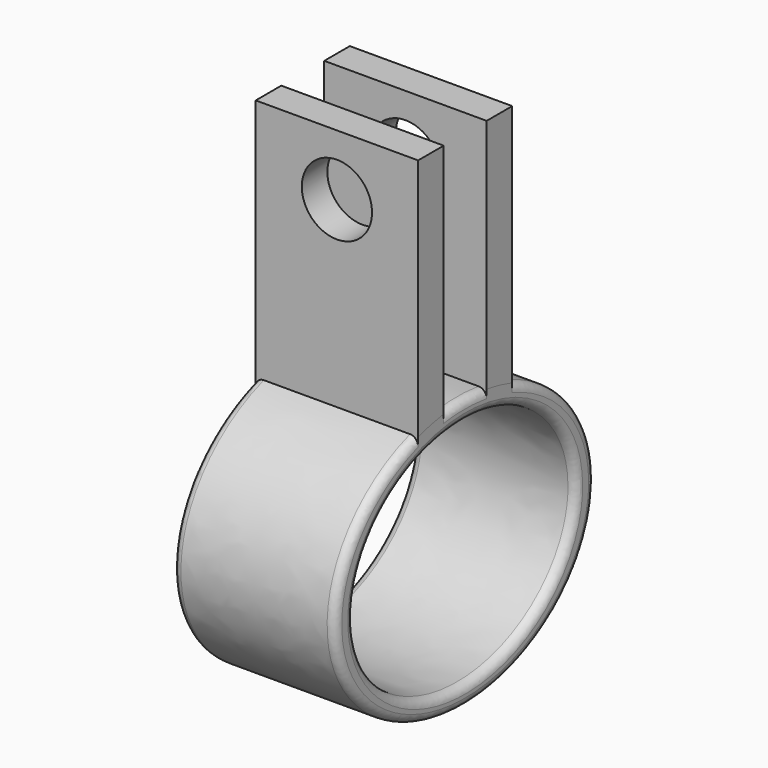
from build123d import *

# Parameters (mm, degrees)
F1_DEPTH = 10.16
F3_DEPTH = 10.16
F4_R     = 2.1971
F5_DEPTH = 25.4
F6_R     = 0.508


with BuildPart() as f1:
    # F0 (on Right) → F1 (new body)
    with BuildSketch(Plane.YZ):
        with BuildLine():
            add(Edge.make_bspline(
                [(10.16, 0), (10.16, 14.6720291858), (-5.08, 7.3360145929), (-20.32, 0), (-5.08, -7.3360145929), (10.16, -14.6720291858), (10.16, 0)],
                knots=[0, 0, 0, 2.0943951024, 2.0943951024, 4.1887902048, 4.1887902048, 6.2831853072, 6.2831853072, 6.2831853072], degree=2, weights=[1, 0.5, 1, 0.5, 1, 0.5, 1]))
        make_face()
        with BuildLine():
            add(Edge.make_bspline(
                [(8.6741, 0), (8.6741, 12.538315796), (-4.33705, 6.269157898), (-17.3482, 0), (-4.33705, -6.269157898), (8.6741, -12.538315796), (8.6741, 0)],
                knots=[0, 0, 0, 2.0943951024, 2.0943951024, 4.1887902048, 4.1887902048, 6.2831853072, 6.2831853072, 6.2831853072], degree=2, weights=[1, 0.5, 1, 0.5, 1, 0.5, 1]))
        make_face(mode=Mode.SUBTRACT)
    extrude(amount=F1_DEPTH)

    # F2 (on face) → F3 (join)
    with BuildSketch(Plane.YZ.offset(10.16)):
        with BuildLine():
            Line((-3.6787074356, 23.1361324366), (-3.6787074356, 7.8961324366))
            add(Edge.make_bspline(
                [(-1.6795329809, 8.3543567658), (-2.7073061404, 8.2107269893), (-3.6787074356, 7.8961324366)],
                knots=[1.698688762, 1.698688762, 1.698688762, 1.9167664316, 1.9167664316, 1.9167664316], degree=2, weights=[0.846760899, 0.8791502713, 0.9223815379]))
            Line((-1.6795329809, 8.3543567658), (-1.6795329809, 23.1361324366))
            Line((-1.6795329809, 23.1361324366), (-3.6787074356, 23.1361324366))
        make_face()
        with BuildLine():
            Line((1.6795329809, 23.1361324366), (1.6795329809, 8.3543567658))
            add(Edge.make_bspline(
                [(3.6787074356, 7.8961324366), (2.7073061404, 8.2107269893), (1.6795329809, 8.3543567658)],
                knots=[1.1863185819, 1.1863185819, 1.1863185819, 1.3749382963, 1.3749382963, 1.3749382963], degree=2, weights=[0.7544123337, 0.7603945573, 0.7744874547]))
            Line((3.6787074356, 7.8961324366), (3.6787074356, 23.1361324366))
            Line((3.6787074356, 23.1361324366), (1.6795329809, 23.1361324366))
        make_face()
    extrude(amount=-F3_DEPTH)

    # F4 (on face) → F5 (cut)
    with BuildSketch(Plane(origin=(0, 3.6787074356, 0), x_dir=(-1, 0, 0), z_dir=(0, 1, 0))):
        with Locations((-5.08, 19.3261324366)):
            Circle(F4_R)
    extrude(amount=-F5_DEPTH, mode=Mode.SUBTRACT)

    # F6
    f6_edges = [f1.edges().sort_by_distance(p)[0] for p in [
        (10.16, -8.6741, 0),
        (10.16, -5.271292, -7.241592),
        (0, -5.271292, -7.241592),
        (0, -8.6741, 0),
        (0, 8.626252, 4.47541),
        (10.16, 8.626252, 4.47541),
        (0, -0.037714, 8.470842),
        (10.16, -0.037714, 8.470842),
    ]]
    fillet(f6_edges, radius=F6_R)


solid = f1.part
